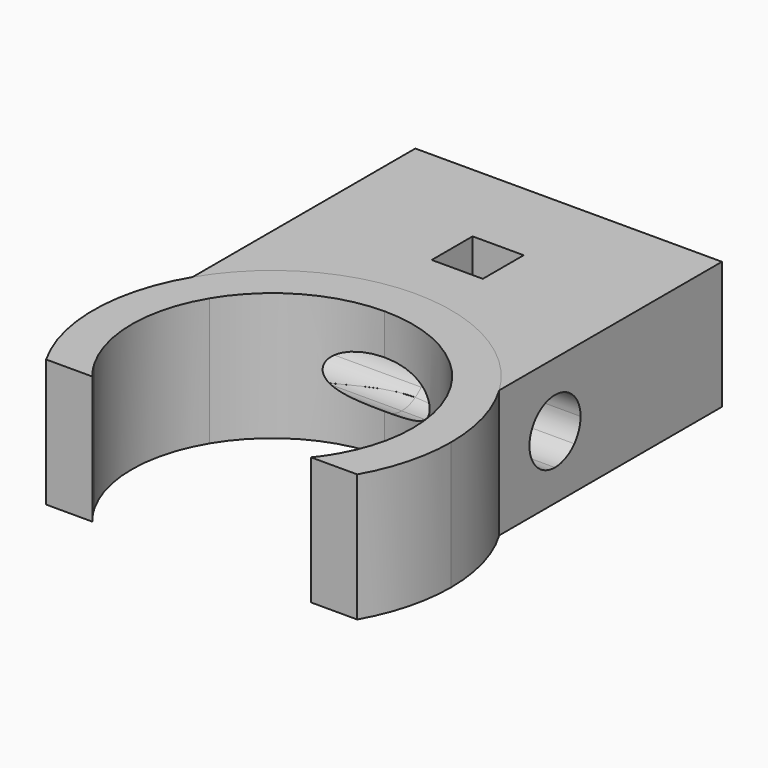
from build123d import *

# Parameters (mm, degrees)
F1_DEPTH      = 10
F2_DEPTH      = 10
F3_T          = -3
F4_DEPTH      = 10
F6_DEPTH      = 25
F6_DEPTH_BACK = 25
F0_W          = 2
F0_H          = 4
F7_DEPTH      = 6


# Not quite as in the source:
# - a feature names something its author has since deleted; it is built from what else it names


with BuildPart() as f1:
    # F0 (on Top) → F1 (new body)
    with BuildSketch(Plane.XY):
        with BuildLine():
            ThreePointArc((12.177598341, -6.9069601595), (13.5367347757, -3.5716679035), (14, 0))
            ThreePointArc((14, 0), (13.4907375632, 3.7416573868), (12, 7.2111025509))
            Line((12, 7.2111025509), (-12, 7.2111025509))
            ThreePointArc((-12, 7.2111025509), (-13.9988924226, 0.1760992369), (-12.177598341, -6.9069601595))
            Line((-12.177598341, -6.9069601595), (12.177598341, -6.9069601595))
        make_face()
        with BuildLine():
            ThreePointArc((-12.177598341, -6.9069601595), (0, -14), (12.177598341, -6.9069601595))
            Line((12.177598341, -6.9069601595), (-12.177598341, -6.9069601595))
        make_face()
        with BuildLine():
            Line((-12, 7.2111025509), (12, 7.2111025509))
            ThreePointArc((12, 7.2111025509), (6.8936407031, 12.1851433252), (0, 14))
            ThreePointArc((0, 14), (-6.8936407031, 12.1851433252), (-12, 7.2111025509))
        make_face()
    extrude(amount=F1_DEPTH)

    # F3
    f3_openings = [f1.faces().sort_by_distance(p)[0] for p in [
        (0, 0, 0),
        (0, 0, 10),
    ]]
    offset(amount=F3_T, openings=f3_openings)

    # F0 (on Top) → F4 (cut)
    with BuildSketch(Plane.XY):
        with BuildLine():
            Line((15.9751549363, -6.9069601595), (12.177598341, -6.9069601595))
            ThreePointArc((12.177598341, -6.9069601595), (0, -14), (-12.177598341, -6.9069601595))
            Line((-12.177598341, -6.9069601595), (-18.203439191, -6.9069601595))
            Line((-18.203439191, -6.9069601595), (-18.203439191, -17.6538378))
            Line((-18.203439191, -17.6538378), (15.9751549363, -17.6538378))
            Line((15.9751549363, -17.6538378), (15.9751549363, -6.9069601595))
        make_face()
        with BuildLine():
            ThreePointArc((-12.177598341, -6.9069601595), (0, -14), (12.177598341, -6.9069601595))
            Line((12.177598341, -6.9069601595), (-12.177598341, -6.9069601595))
        make_face()
    extrude(amount=F4_DEPTH, mode=Mode.SUBTRACT)


with BuildPart() as f2:
    # F0 (on Top) → F2 (new body)
    with BuildSketch(Plane.XY):
        with BuildLine():
            ThreePointArc((-12, 7.2111025509), (-6.8936407031, 12.1851433252), (0, 14))
            Line((0, 14), (0, 18.105))
            Line((0, 18.105), (-2, 18.105))
            Line((-2, 18.105), (-2, 22.105))
            Line((-2, 22.105), (0, 22.105))
            Line((0, 22.105), (0, 29))
            Line((0, 29), (-12, 29))
            Line((-12, 29), (-12, 7.2111025509))
        make_face()
        with BuildLine():
            ThreePointArc((0, 14), (6.8936407031, 12.1851433252), (12, 7.2111025509))
            Line((12, 7.2111025509), (12, 29))
            Line((12, 29), (0, 29))
            Line((0, 29), (0, 22.105))
            Line((0, 22.105), (2, 22.105))
            Line((2, 22.105), (2, 18.105))
            Line((2, 18.105), (0, 18.105))
            Line((0, 18.105), (0, 14))
        make_face()
    extrude(amount=F2_DEPTH)


with BuildPart() as f6_tool:
    # F5 (on Right) → F6 (new body, two sides)
    with BuildSketch(Plane.YZ) as f6_sk:
        with BuildLine():
            ThreePointArc((14.5591712674, 6.5997470737), (13.7068573789, 7.2374578628), (12.6664981618, 7.4627725634))
            Line((12.6664981618, 7.4627725634), (14.5591712674, 6.5997470737))
        make_face()
        with BuildLine():
            ThreePointArc((12.6664981618, 7.4627725634), (10.9007638693, 6.7294296355), (10.1696419809, 4.9627745402))
            Line((10.1696419809, 4.9627745402), (15.1696419809, 4.9627745402))
            ThreePointArc((15.1696419809, 4.9627745402), (15.0120577442, 5.8363238473), (14.5591712674, 6.5997470737))
            Line((14.5591712674, 6.5997470737), (12.6664981618, 7.4627725634))
        make_face()
        with BuildLine():
            ThreePointArc((10.1696419809, 4.9627745402), (10.8995849446, 3.1973006411), (12.6631604515, 2.4627829422))
            Line((12.6631604515, 2.4627829422), (14.5606008683, 3.3274536278))
            ThreePointArc((14.5606008683, 3.3274536278), (15.0124391572, 4.0902486719), (15.1696419809, 4.9627745402))
            Line((15.1696419809, 4.9627745402), (10.1696419809, 4.9627745402))
        make_face()
        with BuildLine():
            Line((14.5606008683, 3.3274536278), (12.6631604515, 2.4627829422))
            ThreePointArc((12.6631604515, 2.4627829422), (13.7063326661, 2.6878520309), (14.5606008683, 3.3274536278))
        make_face()
    extrude(amount=-F6_DEPTH)
    extrude(f6_sk.sketch, amount=F6_DEPTH_BACK)


with BuildPart() as f1_1:
    add(f1.part)

    # F6: cut by f6_tool
    add(f6_tool.part, mode=Mode.SUBTRACT)


with BuildPart() as f2_1:
    add(f2.part)

    # F6: cut by f6_tool
    add(f6_tool.part, mode=Mode.SUBTRACT)

    # F0 (on Top) → F7 (join)
    with BuildSketch(Plane.XY):
        with Locations((1, 20.105)):
            Rectangle(F0_W, F0_H)
        with Locations((-1, 20.105)):
            Rectangle(F0_W, F0_H)
    extrude(amount=F7_DEPTH)


solid = Compound([f1_1.part, f2_1.part])
